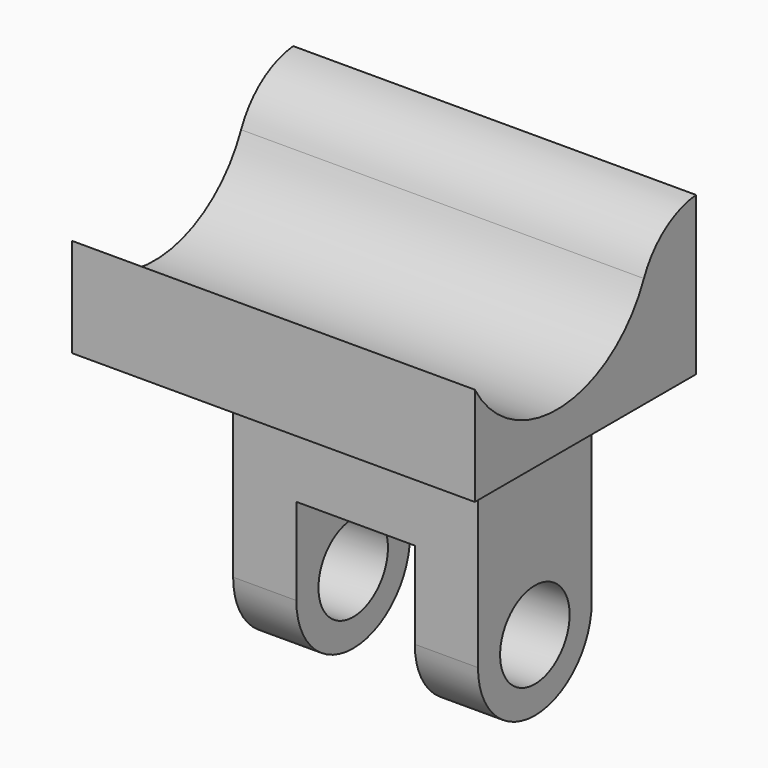
from build123d import *

# Parameters (mm, degrees)
F0_W         = 10.2
F0_H         = 7
F1_DEPTH     = 4
F2_W         = 6.2
F2_H         = 3.6
F3_DEPTH     = 7.2
F4_W         = 3
F4_H         = 4
F5_DEPTH     = 25
F6_R         = 1.79999
F7_R         = 1.1
F8_DEPTH     = 25
F9_R         = 3
F10_DEPTH    = 25
F11_T1_DEPTH = 17.2


# Not quite as in the source:
# - a fillet or chamfer that OpenCascade refuses, or shapes differently, is made with other operations: its cross-section is extruded or revolved along the edge and cut away or added
# - a fillet or chamfer is up to 0.001 mm smaller than in the source, because OpenCascade refuses the exact size


with BuildPart() as f1:
    # F0 (on Top) → F1 (new body)
    with BuildSketch(Plane.XY):
        with Locations((5.1, 3.5)):
            Rectangle(F0_W, F0_H)
    extrude(amount=F1_DEPTH)

    # F2 (on face) → F3 (join)
    with BuildSketch(Plane(origin=(0, 0, 0), x_dir=(1, 0, 0), z_dir=(0, 0, -1))):
        with Locations((5.1, -4.4)):
            Rectangle(F2_W, F2_H)
    extrude(amount=F3_DEPTH)

    # F4 (on face) → F5 (cut)
    with BuildSketch(Plane(origin=(0, 6.2, 0), x_dir=(-1, 0, 0), z_dir=(0, 1, 0))):
        with Locations((-5.1, -5.2)):
            Rectangle(F4_W, F4_H)
    extrude(amount=-F5_DEPTH, mode=Mode.SUBTRACT)

    # F6 (radius 1.8 in the source; OpenCascade refuses exactly that, so slightly less here)
    f6_edges = [f1.edges().sort_by_distance(p)[0] for p in [
        (2.8, 2.6, -7.2),
        (7.4, 2.6, -7.2),
        (2.8, 6.2, -7.2),
        (7.4, 6.2, -7.2),
    ]]
    fillet(f6_edges, radius=F6_R)

    # F7 (on face) → F8 (cut)
    with BuildSketch(Plane.YZ.offset(8.2)):
        with Locations((4.4, -5.4)):
            Circle(F7_R)
    extrude(amount=-F8_DEPTH, mode=Mode.SUBTRACT)

    # F9 (on face) → F10 (cut)
    with BuildSketch(Plane(origin=(0, 0, 0), x_dir=(0, -1, 0), z_dir=(-1, 0, 0))):
        with Locations((-2.6, 4)):
            Circle(F9_R)
    extrude(amount=-F10_DEPTH, mode=Mode.SUBTRACT)

    # F11: fillet of radius 2 on 1 edges, made by hand

    # F11_s2 → F11_t1 (cut)
    with BuildSketch(Plane.YZ.offset(-3.5)):
        with BuildLine():
            ThreePointArc((5.3518181818, 2.8052210689), (6.0125269518, 3.627994046), (7, 4))
            Line((7, 4), (5.6, 4))
            ThreePointArc((5.6, 4), (5.5372993162, 3.3898584367), (5.3518181818, 2.8052210689))
        make_face()
    extrude(amount=F11_T1_DEPTH, mode=Mode.SUBTRACT)


solid = f1.part
